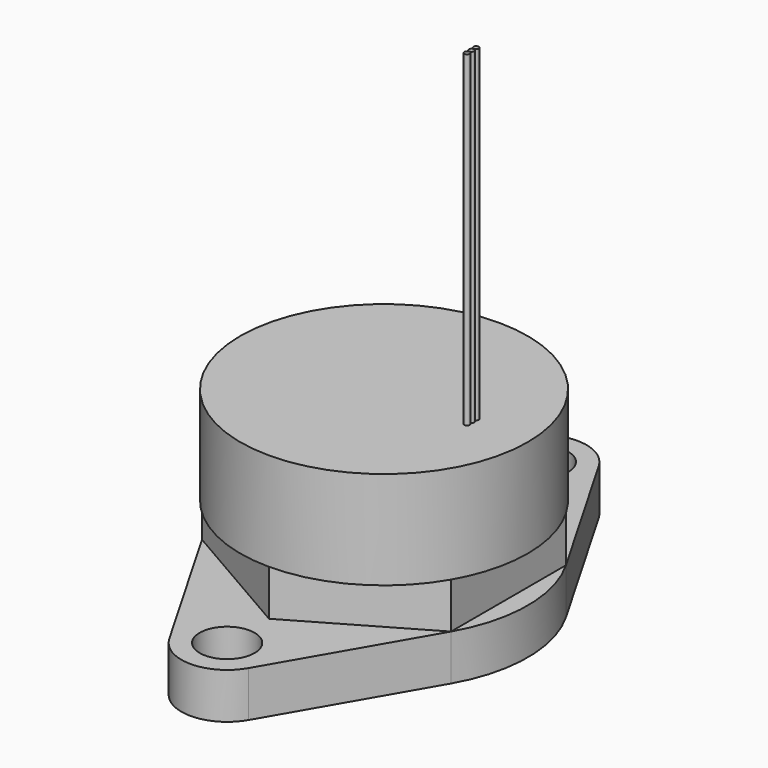
from build123d import *

# Parameters (mm, degrees)
F0_R      = 11
F1_DEPTH  = 14.5
F2_R      = 2.1
F3_DEPTH  = 3.5
F4_R      = 11
F5_DEPTH  = 3.5
F7_DEPTH  = 3.5
F8_R      = 6.5
F9_DEPTH  = 7.87
F10_R     = 0.2032
F11_DEPTH = 25


# Not quite as in the source:
# - a pattern or mirror of a feature is missing from the dataset's text; its kind, count and spacing are read off the source's solid


with BuildPart() as f1:
    # F0 (on Top) → F1 (new body)
    with BuildSketch(Plane.XY):
        Circle(F0_R)
    extrude(amount=F1_DEPTH)

    # F2 (on face) → F3 (join)
    with BuildSketch(Plane(origin=(0, 0, 0), x_dir=(1, 0, 0), z_dir=(0, 0, -1))):
        with BuildLine():
            Line((9.5262794416, 5.5), (3.0310889132, 16.75))
            ThreePointArc((3.0310889132, 16.75), (0, 18.5), (-3.0310889132, 16.75))
            Line((-3.0310889132, 16.75), (-9.5262794416, 5.5))
            ThreePointArc((-9.5262794416, 5.5), (0, 11), (9.5262794416, 5.5))
        make_face()
        with Locations((0, 15)):
            Circle(F2_R, mode=Mode.SUBTRACT)
        with BuildLine():
            ThreePointArc((9.5262794416, -5.5), (0, -11), (-9.5262794416, -5.5))
            Line((-9.5262794416, -5.5), (-3.0310889132, -16.75))
            ThreePointArc((-3.0310889132, -16.75), (0, -18.5), (3.0310889132, -16.75))
            Line((3.0310889132, -16.75), (9.5262794416, -5.5))
        make_face()
        with Locations((0, -15)):
            Circle(F2_R, mode=Mode.SUBTRACT)
    f3 = extrude(amount=-F3_DEPTH)

    # F3_copies: F3 across plane
    add(f3.mirror(Plane(origin=(0, 0, 0), x_dir=(0, 0, -1), z_dir=(-1, 0, 0))))

    # F4 (on face) → F5 (cut)
    with BuildSketch(Plane.XY.offset(3.5)):
        Circle(F4_R)
    extrude(amount=F5_DEPTH, mode=Mode.SUBTRACT)

    # F6 (on face) → F7 (join)
    with BuildSketch(Plane.XY.offset(3.5)):
        Polygon((9.5262794416, 5.5), (0, 11), (-9.5262794416, 5.5), (-9.5262794416, -5.5), (0, -11), (9.5262794416, -5.5), align=None)
    extrude(amount=F7_DEPTH)

    # F8 (on face) → F9 (cut)
    with BuildSketch(Plane(origin=(0, 0, 0), x_dir=(1, 0, 0), z_dir=(0, 0, -1))):
        Circle(F8_R)
    extrude(amount=-F9_DEPTH, mode=Mode.SUBTRACT)

    # F10 (on face) → F11 (join)
    with BuildSketch(Plane.XY.offset(14.5)):
        with Locations((6.7, 0)):
            Circle(F10_R)
        with Locations((6.7, 0.4318)):
            Circle(F10_R)
        with Locations((6.7, -0.4318)):
            Circle(F10_R)
    extrude(amount=F11_DEPTH)


solid = f1.part
